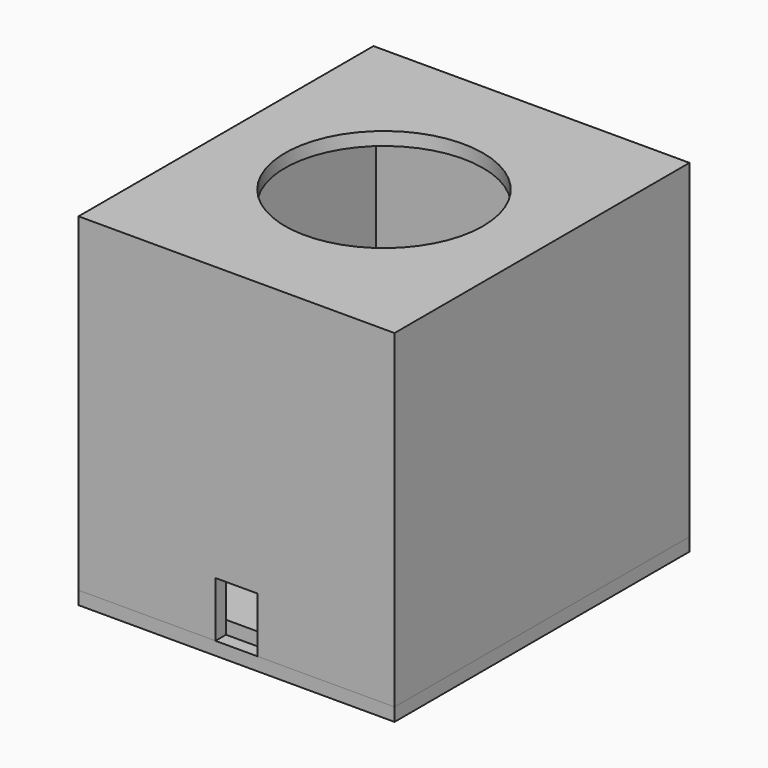
from build123d import *

# Parameters (mm, degrees)
F0_W     = 38.1
F0_H     = 44.45
F0_R     = 11.938
F1_DEPTH = 1.5875
F2_W     = 38.1
F2_H     = 44.45
F2_W_2   = 34.925
F2_H_2   = 41.275
F3_DEPTH = 38.1
F4_W     = 5.08
F4_H     = 6.6675
F5_DEPTH = 1.5875
F7_DEPTH = 1.5875
F8_W     = 34.925
F8_H     = 41.275
F9_DEPTH = 1.5875


with BuildPart() as f1:
    # F0 (on Top) → F1 (new body)
    with BuildSketch(Plane.XY):
        Rectangle(F0_W, F0_H)
        Circle(F0_R, mode=Mode.SUBTRACT)
    extrude(amount=-F1_DEPTH)

    # F2 (on face) → F3 (join)
    with BuildSketch(Plane(origin=(0, 0, -1.5875), x_dir=(1, 0, 0), z_dir=(0, 0, -1))):
        Rectangle(F2_W, F2_H)
        Rectangle(F2_W_2, F2_H_2, mode=Mode.SUBTRACT)
    extrude(amount=F3_DEPTH)

    # F4 (on face) → F5 (cut, through all)
    with BuildSketch(Plane.XZ.offset(22.225)):
        with Locations((0, -36.35375)):
            Rectangle(F4_W, F4_H)
    extrude(amount=-F5_DEPTH, mode=Mode.SUBTRACT)


with BuildPart() as f7:
    # F6 (on face) → F7 (new body)
    with BuildSketch(Plane(origin=(0, 0, -39.6875), x_dir=(1, 0, 0), z_dir=(0, 0, -1))):
        Polygon((19.05, 22.225), (2.54, 22.225), (-2.54, 22.225), (-19.05, 22.225), (-19.05, -22.225), (19.05, -22.225), align=None)
    extrude(amount=F7_DEPTH)

    # F8 (on face) → F9 (join)
    with BuildSketch(Plane.XY.offset(-39.6875)):
        Rectangle(F8_W, F8_H)
    extrude(amount=F9_DEPTH)


solid = Compound([f1.part, f7.part])
